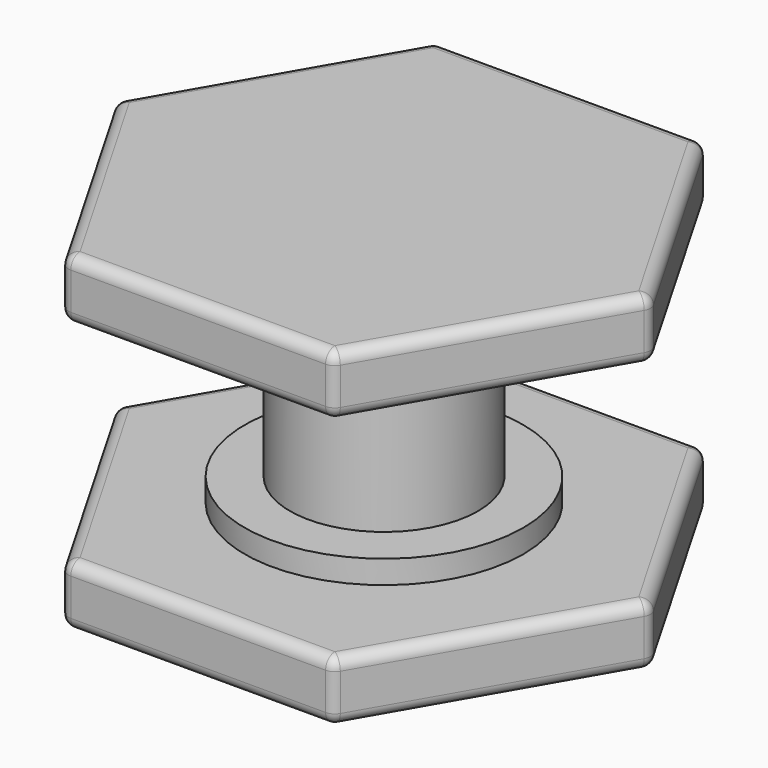
from build123d import *

# Parameters (mm, degrees)
F0_R      = 6
F0_R_2    = 4.05
F1_DEPTH  = 1
F2_DEPTH  = 7
F4_DEPTH  = 2.6
F5_R      = 6
F5_R_2    = 4.05
F6_DEPTH  = 1
F8_DEPTH  = 2.6
F9_R      = 0.5
F9_2_R    = 0.5
F10_R     = 2.25
F11_DEPTH = 7
F14_R     = 2.25
F15_DEPTH = 7


with BuildPart() as f1:
    # F0 (on Top) → F1 (new body)
    with BuildSketch(Plane.XY):
        Circle(F0_R)
        Circle(F0_R_2, mode=Mode.SUBTRACT)
        Circle(F0_R_2)
    extrude(amount=F1_DEPTH)

    # F0 (on Top) → F2 (join)
    with BuildSketch(Plane.XY):
        Circle(F0_R_2)
    extrude(amount=-F2_DEPTH)

    # F3 (on face) → F4 (join)
    with BuildSketch(Plane.XY.offset(1)):
        Polygon((-5.7735026919, -10), (5.7735026919, -10), (11.5470053838, 0), (5.7735026919, 10), (-5.7735026919, 10), (-11.5470053838, 0), align=None)
    extrude(amount=F4_DEPTH)

    # F9
    f9_edges = [f1.edges().sort_by_distance(p)[0] for p in [
        (5.773503, -10, 2.3),
        (11.547005, 0, 2.3),
        (8.660254, -5, 1),
        (8.660254, -5, 3.6),
        (5.773503, 10, 2.3),
        (8.660254, 5, 1),
        (8.660254, 5, 3.6),
        (-5.773503, -10, 2.3),
        (0, -10, 1),
        (0, -10, 3.6),
        (-11.547005, 0, 2.3),
        (-8.660254, -5, 1),
        (-8.660254, -5, 3.6),
        (-5.773503, 10, 2.3),
        (-8.660254, 5, 1),
        (-8.660254, 5, 3.6),
        (0, 10, 1),
        (0, 10, 3.6),
    ]]
    fillet(f9_edges, radius=F9_R)

    # F10 (on face) → F11 (cut)
    with BuildSketch(Plane(origin=(0, 0, -7), x_dir=(1, 0, 0), z_dir=(0, 0, -1))):
        Circle(F10_R)
    extrude(amount=-F11_DEPTH, mode=Mode.SUBTRACT)

    # F12 (on Right) → F13 (revolve, cut)
    with BuildSketch(Plane.YZ):
        with BuildLine():
            Line((2.25, 0), (2.25, -0.996934039))
            ThreePointArc((2.25, -0.996934039), (2.3830913367, -0.4984670195), (2.25, 0))
        make_face()
    revolve(axis=Axis((0, 0, -3.8720492739), (0, 0, -1)), mode=Mode.SUBTRACT)


with BuildPart() as f6:
    # F5 (on face) → F6 (new body)
    with BuildSketch(Plane(origin=(0, 0, -7), x_dir=(1, 0, 0), z_dir=(0, 0, -1))):
        Circle(F5_R)
        Circle(F5_R_2, mode=Mode.SUBTRACT)
        Circle(F5_R_2)
    extrude(amount=F6_DEPTH)

    # F7 (on face) → F8 (join)
    with BuildSketch(Plane(origin=(0, 0, -8), x_dir=(1, 0, 0), z_dir=(0, 0, -1))):
        Polygon((5.7735026919, -10), (11.5470053838, 0), (5.7735026919, 10), (-5.7735026919, 10), (-11.5470053838, 0), (-5.7735026919, -10), align=None)
    extrude(amount=F8_DEPTH)

    # F9#2
    f9_2_edges = [f6.edges().sort_by_distance(p)[0] for p in [
        (5.773503, -10, -9.3),
        (-5.773503, -10, -9.3),
        (0, -10, -8),
        (0, -10, -10.6),
        (11.547005, 0, -9.3),
        (8.660254, -5, -8),
        (8.660254, -5, -10.6),
        (5.773503, 10, -9.3),
        (8.660254, 5, -8),
        (8.660254, 5, -10.6),
        (-5.773503, 10, -9.3),
        (0, 10, -8),
        (0, 10, -10.6),
        (-11.547005, 0, -9.3),
        (-8.660254, 5, -8),
        (-8.660254, 5, -10.6),
        (-8.660254, -5, -8),
        (-8.660254, -5, -10.6),
    ]]
    fillet(f9_2_edges, radius=F9_2_R)

    # F14 (on face) → F15 (join, through all)
    with BuildSketch(Plane.XY.offset(-7)):
        Circle(F14_R)
    extrude(amount=F15_DEPTH)

    # F16 (on Right) → F17 (revolve)
    with BuildSketch(Plane.YZ):
        with BuildLine():
            Line((-2.2414149716, -0.9849705966), (-2.2414149716, 0))
            ThreePointArc((-2.2414149716, 0), (-2.3471306252, -0.4924852983), (-2.2414149716, -0.9849705966))
        make_face()
    revolve(axis=Axis((0, 0, -3.7047876976), (0, 0, -1)))


solid = Compound([f1.part, f6.part])
